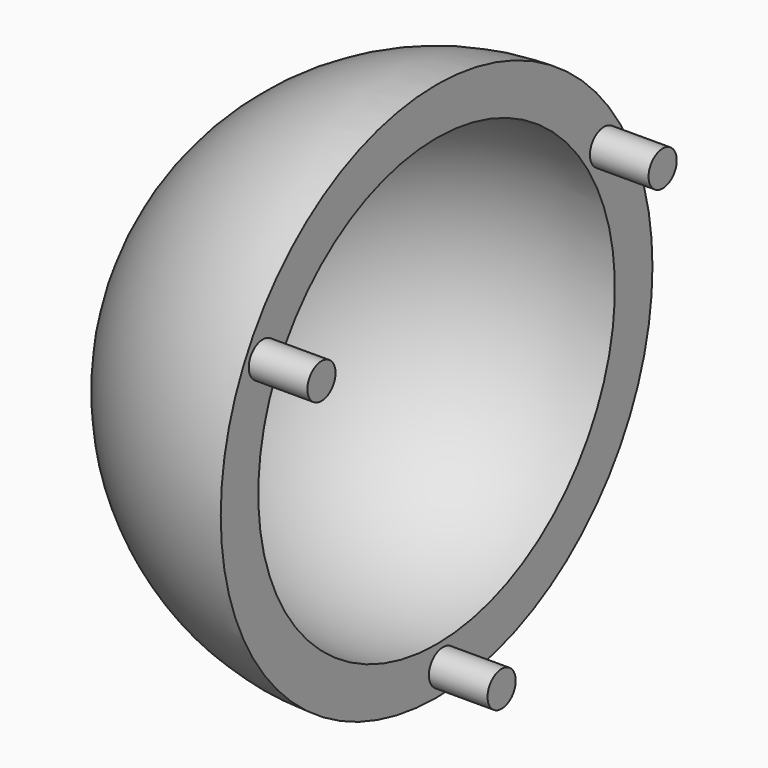
from build123d import *

# Parameters (mm, degrees)
F2_W            = 26.7493221909
F2_H            = 40.8729631454
F3_DEPTH        = 25
F3_DEPTH_BACK   = 37.9
F6_R            = 0.75
F7_DEPTH        = 2.5
F7_COPIES_COUNT = 3


# Not quite as in the source:
# - a pattern or mirror of a feature is missing from the dataset's text; its kind, count and spacing are read off the source's solid


with BuildPart() as f1:
    # F0 (on Top) → F1 (revolve)
    with BuildSketch(Plane.XY):
        with BuildLine():
            Line((0, 11.5), (0, -11.5))
            ThreePointArc((0, -11.5), (11.5, 0), (0, 11.5))
        make_face()
    revolve(axis=Axis((0, 0, 0), (0, -1, 0)))

    # F2 (on Top) → F3 (cut, two sides)
    with BuildSketch(Plane.XY) as f3_sk:
        with Locations((13.3746610954, -0.1069968566)):
            Rectangle(F2_W, F2_H)
    extrude(amount=-F3_DEPTH, mode=Mode.SUBTRACT)
    extrude(f3_sk.sketch, amount=F3_DEPTH_BACK, mode=Mode.SUBTRACT)

    # F4 (on face) → F5 (revolve, cut)
    with BuildSketch(Plane.YZ):
        with BuildLine():
            Line((0, 9.5), (0, -9.5))
            ThreePointArc((0, -9.5), (9.5, 0), (0, 9.5))
        make_face()
    revolve(axis=Axis((0, 0, 0), (0, 0, -1)), mode=Mode.SUBTRACT)

    # F6 (on face) → F7 (join)
    with BuildSketch(Plane.YZ):
        with Locations((-9.2580689408, 4.9536006588)):
            Circle(F6_R)
    f7 = extrude(amount=F7_DEPTH)

    # F7_copies: F7 ×3 about axis
    f7_copies_axis = Axis((0, 0, 0), (1, 0, 0))
    for i in range(1, F7_COPIES_COUNT):
        add(f7.rotate(f7_copies_axis, i * 360 / F7_COPIES_COUNT))


solid = f1.part
